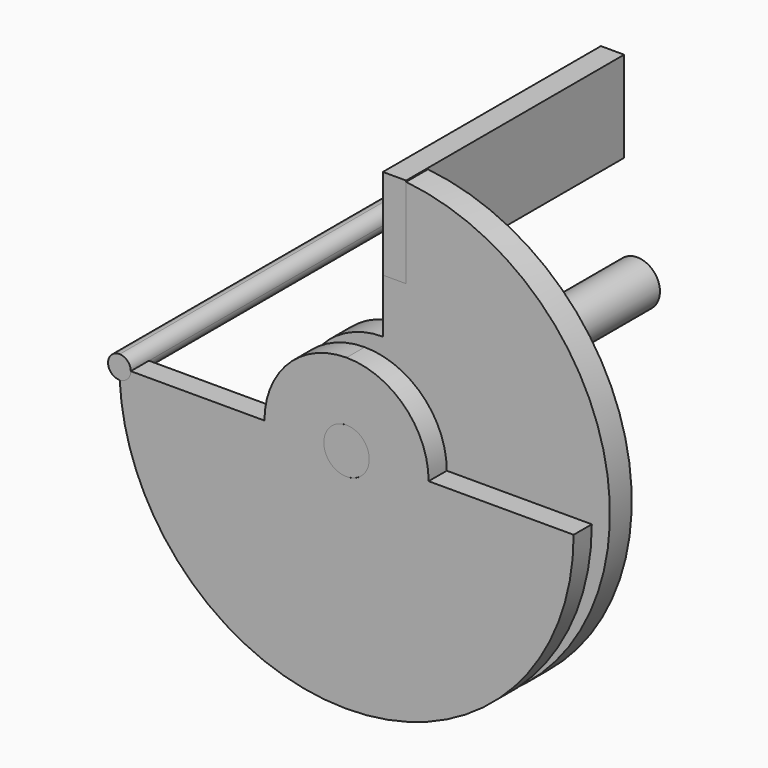
from build123d import *

# Parameters (mm, degrees)
F0_R     = 3.175
F1_DEPTH = 25.4
F2_DEPTH = 19.05
F4_DEPTH = 3.81
F6_DEPTH = 3.175


with BuildPart() as f1:
    # F0 (on Front) → F1 (new body, symmetric)
    with BuildSketch(Plane.XZ):
        Circle(F0_R)
    extrude(amount=F1_DEPTH, both=True)


with BuildPart() as f1b:
    # F0 (on Front) → F1, piece 2 (new body, symmetric)
    with BuildSketch(Plane.XZ):
        with BuildLine():
            ThreePointArc((-31.710313, 1.587004), (-33.3375, 0), (-31.710313, -1.587004))
            ThreePointArc((-31.710313, -1.587004), (-31.75, 0), (-31.710313, 1.587004))
        make_face()
        with BuildLine():
            ThreePointArc((-31.710313, 1.587004), (-31.75, 0), (-31.710313, -1.587004))
            ThreePointArc((-31.710313, -1.587004), (-30.613523, -1.108412), (-30.1625, 0))
            ThreePointArc((-30.1625, 0), (-30.613523, 1.108412), (-31.710313, 1.587004))
        make_face()
    extrude(amount=F1_DEPTH, both=True)


with BuildPart() as f2:
    # F0 (on Front) → F2 (new body, symmetric)
    with BuildSketch(Plane.XZ):
        with BuildLine():
            ThreePointArc((0, 31.75), (1.627741, 31.708248), (3.2512, 31.5831))
            Line((3.2512, 31.5831), (3.2512, 31.75))
            Line((3.2512, 31.75), (0, 31.75))
        make_face()
        with BuildLine():
            Line((3.2512, 19.05), (3.2512, 31.5831))
            ThreePointArc((3.2512, 31.5831), (1.627741, 31.708248), (0, 31.75))
            Line((0, 31.75), (0, 19.05))
            Line((0, 19.05), (3.2512, 19.05))
        make_face()
    extrude(amount=F2_DEPTH, both=True)


with BuildPart() as f4:
    # F3 (on face) → F4 (new body)
    with BuildSketch(Plane.XZ.offset(19.05)):
        with BuildLine():
            Line((3.2512, 31.5831), (3.2512, 19.05))
            Line((3.2512, 19.05), (0, 19.05))
            Line((0, 19.05), (0, 11.476406))
            Line((0, 11.476406), (0, 3.175))
            ThreePointArc((0, 3.175), (2.245064, 2.245064), (3.175, 0))
            ThreePointArc((3.175, 0), (1.385946, -2.856533), (-1.965019, -2.493858))
            Line((-1.965019, -2.493858), (-8.845686, -7.311753))
            Line((-8.845686, -7.311753), (-25.471999, -18.953622))
            ThreePointArc((-25.471999, -18.953622), (27.603098, -15.688577), (3.2512, 31.5831))
        make_face()
        with BuildLine():
            Line((0, 3.175), (0, 11.476406))
            ThreePointArc((0, 11.476406), (-10.383172, 4.88852), (-8.845686, -7.311753))
            Line((-8.845686, -7.311753), (-1.965019, -2.493858))
            ThreePointArc((-1.965019, -2.493858), (-2.999885, 1.039862), (0, 3.175))
        make_face()
    extrude(amount=-F4_DEPTH)


with BuildPart() as f6:
    # F5 (on face) → F6 (new body)
    with BuildSketch(Plane.XZ.offset(25.4)):
        with BuildLine():
            ThreePointArc((-31.710312, -1.587004), (-29.880663, -10.733521), (-25.471999, -18.953622))
            Line((-25.471999, -18.953622), (-8.845686, -7.311753))
            ThreePointArc((-8.845686, -7.311753), (-10.798717, -3.885306), (-11.476406, 0))
            Line((-11.476406, 0), (-30.1625, 0))
            ThreePointArc((-30.1625, 0), (-30.613523, -1.108412), (-31.710312, -1.587004))
        make_face()
        with BuildLine():
            ThreePointArc((-11.476406, 0), (-10.798717, -3.885306), (-8.845686, -7.311753))
            Line((-8.845686, -7.311753), (-1.965019, -2.493858))
            ThreePointArc((-1.965019, -2.493858), (-2.856533, -1.385946), (-3.175, 0))
            Line((-3.175, 0), (-11.476406, 0))
        make_face()
        with BuildLine():
            Line((-1.965019, -2.493858), (-8.845686, -7.311753))
            ThreePointArc((-8.845686, -7.311753), (3.885306, -10.798717), (11.476406, 0))
            Line((11.476406, 0), (3.175, 0))
            ThreePointArc((3.175, 0), (1.385946, -2.856533), (-1.965019, -2.493858))
        make_face()
        with BuildLine():
            ThreePointArc((0, 11.476406), (-8.115044, 8.115044), (-11.476406, 0))
            Line((-11.476406, 0), (-3.175, 0))
            ThreePointArc((-3.175, 0), (-2.245064, 2.245064), (0, 3.175))
            Line((0, 3.175), (0, 11.476406))
        make_face()
        with BuildLine():
            Line((3.175, 0), (11.476406, 0))
            ThreePointArc((11.476406, 0), (8.115044, 8.115044), (0, 11.476406))
            Line((0, 11.476406), (0, 3.175))
            ThreePointArc((0, 3.175), (2.245064, 2.245064), (3.175, 0))
        make_face()
        with BuildLine():
            Line((-8.845686, -7.311753), (-25.471999, -18.953622))
            ThreePointArc((-25.471999, -18.953622), (9.983149, -30.139662), (31.75, 0))
            Line((31.75, 0), (11.476406, 0))
            ThreePointArc((11.476406, 0), (3.885306, -10.798717), (-8.845686, -7.311753))
        make_face()
    extrude(amount=-F6_DEPTH)


solid = Compound([f1.part, f1b.part, f2.part, f4.part, f6.part])
